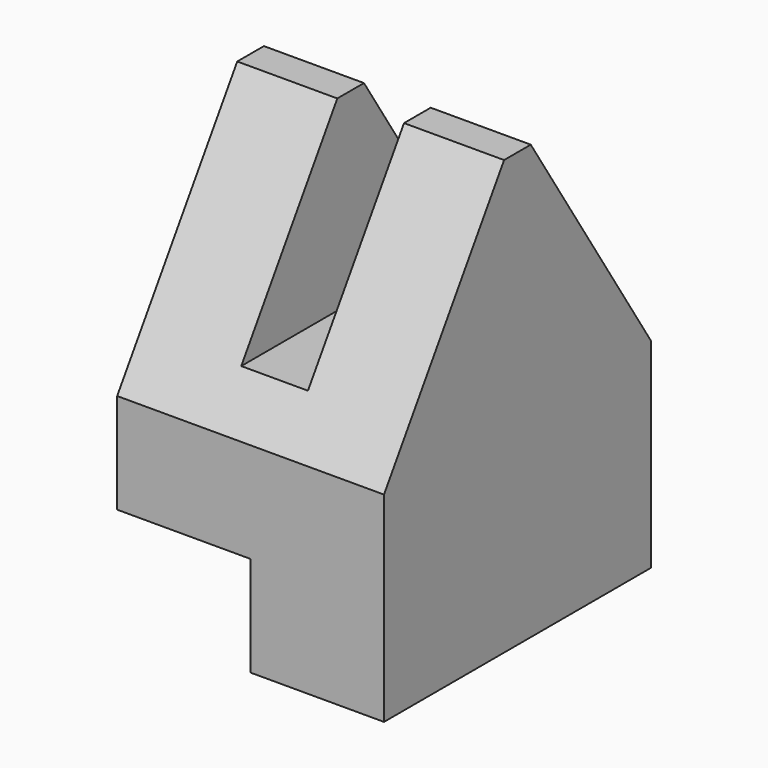
from build123d import *

# Parameters (mm, degrees)
F1_DEPTH = 20
F2_W     = 20
F2_H     = 15
F3_DEPTH = 50.001
F4_W     = 10
F4_H     = 22.5
F4_H_2   = 5
F5_DEPTH = 28


with BuildPart() as f1:
    # F0 (on Right) → F1 (new body, symmetric)
    with BuildSketch(Plane.YZ):
        Polygon((-25, 15), (0, 15), (0, 50), (-2.5, 50), align=None)
        Polygon((25, -15), (25, 15), (0, 15), (-25, 15), (-25, -15), align=None)
        Polygon((0, 15), (25, 15), (2.5, 50), (0, 50), align=None)
    extrude(amount=F1_DEPTH, both=True)

    # F2 (on face) → F3 (cut, through all)
    with BuildSketch(Plane.XZ.offset(25)):
        with Locations((-10, -7.5)):
            Rectangle(F2_W, F2_H)
    extrude(amount=-F3_DEPTH, mode=Mode.SUBTRACT)

    # F4 (on face) → F5 (cut)
    with BuildSketch(Plane.XY.offset(50)):
        with Locations((0, -13.75)):
            Rectangle(F4_W, F4_H)
        Rectangle(F4_W, F4_H_2)
        with Locations((0, 13.75)):
            Rectangle(F4_W, F4_H)
    extrude(amount=-F5_DEPTH, mode=Mode.SUBTRACT)


solid = f1.part
